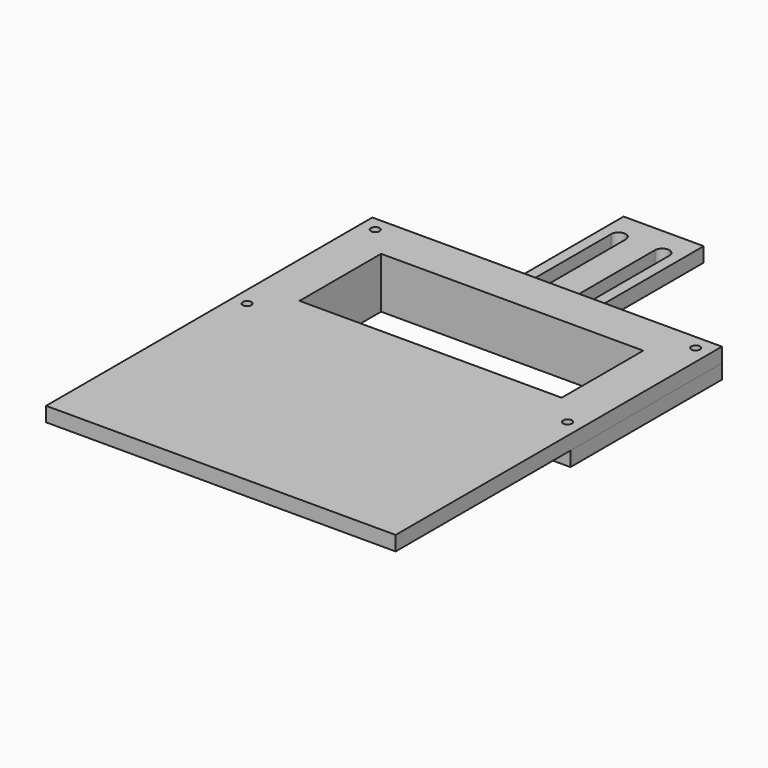
from build123d import *

# Parameters (mm, degrees)
F1_R          = 3
F1_W          = 190
F1_H          = 80
F2_DEPTH      = 10
F1_W_2        = 180
F1_H_2        = 70
F3_DEPTH      = 5
F4_START      = 10
F1_W_3        = 240
F1_H_3        = 150
F4_DEPTH      = 10
F5_DEPTH      = 20
F5_DEPTH_BACK = 15


with BuildPart() as f2:
    # F1 (on Top) → F2 (new body)
    with BuildSketch(Plane.XY):
        with BuildLine():
            ThreePointArc((292.5, 333), (291.6213203436, 330.8786796564), (289.5, 330))
            Line((289.5, 330), (350.5, 330))
            ThreePointArc((350.5, 330), (348.3786796564, 330.8786796564), (347.5, 333))
            Line((347.5, 333), (347.5, 430))
            Line((347.5, 430), (292.5, 430))
            Line((292.5, 430), (292.5, 333))
        make_face()
        with BuildLine():
            Line((300, 345), (300, 410))
            ThreePointArc((300, 410), (305, 415), (310, 410))
            Line((310, 410), (310, 345))
            ThreePointArc((310, 345), (305, 340), (300, 345))
        make_face(mode=Mode.SUBTRACT)
        with BuildLine():
            Line((330, 345), (330, 410))
            ThreePointArc((330, 410), (335, 415), (340, 410))
            Line((340, 410), (340, 345))
            ThreePointArc((340, 345), (335, 340), (330, 345))
        make_face(mode=Mode.SUBTRACT)
        Polygon((200, 330), (200, 200), (440, 200), (440, 330), (350.5, 330), (289.5, 330), align=None)
        with Locations((210, 210)):
            Circle(F1_R, mode=Mode.SUBTRACT)
        with Locations((430, 210)):
            Circle(F1_R, mode=Mode.SUBTRACT)
        with Locations((210, 320)):
            Circle(F1_R, mode=Mode.SUBTRACT)
        with Locations((320, 265)):
            Rectangle(F1_W, F1_H, mode=Mode.SUBTRACT)
        with Locations((430, 320)):
            Circle(F1_R, mode=Mode.SUBTRACT)
    extrude(amount=F2_DEPTH)

    # F1 (on Top) → F3 (join)
    with BuildSketch(Plane.XY):
        with BuildLine():
            ThreePointArc((292.5, 333), (291.6213203436, 330.8786796564), (289.5, 330))
            Line((289.5, 330), (350.5, 330))
            ThreePointArc((350.5, 330), (348.3786796564, 330.8786796564), (347.5, 333))
            Line((347.5, 333), (347.5, 430))
            Line((347.5, 430), (292.5, 430))
            Line((292.5, 430), (292.5, 333))
        make_face()
        with BuildLine():
            Line((300, 345), (300, 410))
            ThreePointArc((300, 410), (305, 415), (310, 410))
            Line((310, 410), (310, 345))
            ThreePointArc((310, 345), (305, 340), (300, 345))
        make_face(mode=Mode.SUBTRACT)
        with BuildLine():
            Line((330, 345), (330, 410))
            ThreePointArc((330, 410), (335, 415), (340, 410))
            Line((340, 410), (340, 345))
            ThreePointArc((340, 345), (335, 340), (330, 345))
        make_face(mode=Mode.SUBTRACT)
        Polygon((200, 330), (200, 200), (440, 200), (440, 330), (350.5, 330), (289.5, 330), align=None)
        with Locations((210, 210)):
            Circle(F1_R, mode=Mode.SUBTRACT)
        with Locations((430, 210)):
            Circle(F1_R, mode=Mode.SUBTRACT)
        with Locations((210, 320)):
            Circle(F1_R, mode=Mode.SUBTRACT)
        with Locations((320, 265)):
            Rectangle(F1_W, F1_H, mode=Mode.SUBTRACT)
        with Locations((430, 320)):
            Circle(F1_R, mode=Mode.SUBTRACT)
        with Locations((320, 265)):
            Rectangle(F1_W, F1_H)
        with Locations((320, 265)):
            Rectangle(F1_W_2, F1_H_2, mode=Mode.SUBTRACT)
    extrude(amount=F3_DEPTH)


with BuildPart() as f4:
    # F1 (on Top) → F4 (new body)
    with BuildSketch(Plane.XY.offset(F4_START)):
        Polygon((200, 330), (200, 200), (440, 200), (440, 330), (350.5, 330), (289.5, 330), align=None)
        with Locations((210, 210)):
            Circle(F1_R, mode=Mode.SUBTRACT)
        with Locations((430, 210)):
            Circle(F1_R, mode=Mode.SUBTRACT)
        with Locations((210, 320)):
            Circle(F1_R, mode=Mode.SUBTRACT)
        with Locations((320, 265)):
            Rectangle(F1_W, F1_H, mode=Mode.SUBTRACT)
        with Locations((430, 320)):
            Circle(F1_R, mode=Mode.SUBTRACT)
        with Locations((320, 125)):
            Rectangle(F1_W_3, F1_H_3)
    extrude(amount=F4_DEPTH)

    # F1 (on Top) → F5 (join, two sides)
    with BuildSketch(Plane.XY) as f5_sk:
        with Locations((320, 265)):
            Rectangle(F1_W, F1_H)
        with Locations((320, 265)):
            Rectangle(F1_W_2, F1_H_2, mode=Mode.SUBTRACT)
    extrude(amount=F5_DEPTH)
    extrude(f5_sk.sketch, amount=-F5_DEPTH_BACK)


solid = Compound([f2.part, f4.part])
